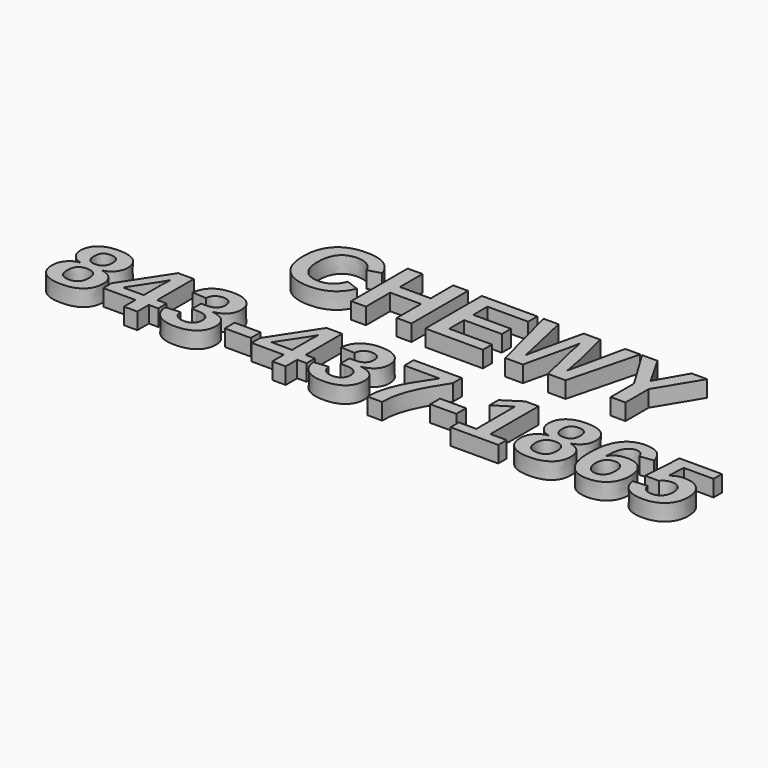
from build123d import *

# Parameters (mm, degrees)
F4_TEXT_SIZE = 6.25
F5_DEPTH     = 1


# Not quite as in the source:
# - Text() gives the source's letters only with a copy of the font that has no kerning and outlines rounded to 1/6400 em; it was checked with that copy


with BuildPart() as f5:
    # F4 (on offset) → F5 (new body)
    with BuildSketch(Plane.XY.offset(14)):
        with Locations((-10.9939306212, 2.3501984853)):
            Text('CHEWY', F4_TEXT_SIZE, font='Arimo', font_style=FontStyle.BOLD, text_align=(TextAlign.LEFT, TextAlign.BOTTOM))
        with Locations((-19.6755712462, -4.8373015147)):
            Text('843-437-1865', F4_TEXT_SIZE, font='Arimo', font_style=FontStyle.BOLD, text_align=(TextAlign.LEFT, TextAlign.BOTTOM))
    extrude(amount=F5_DEPTH)


solid = f5.part
